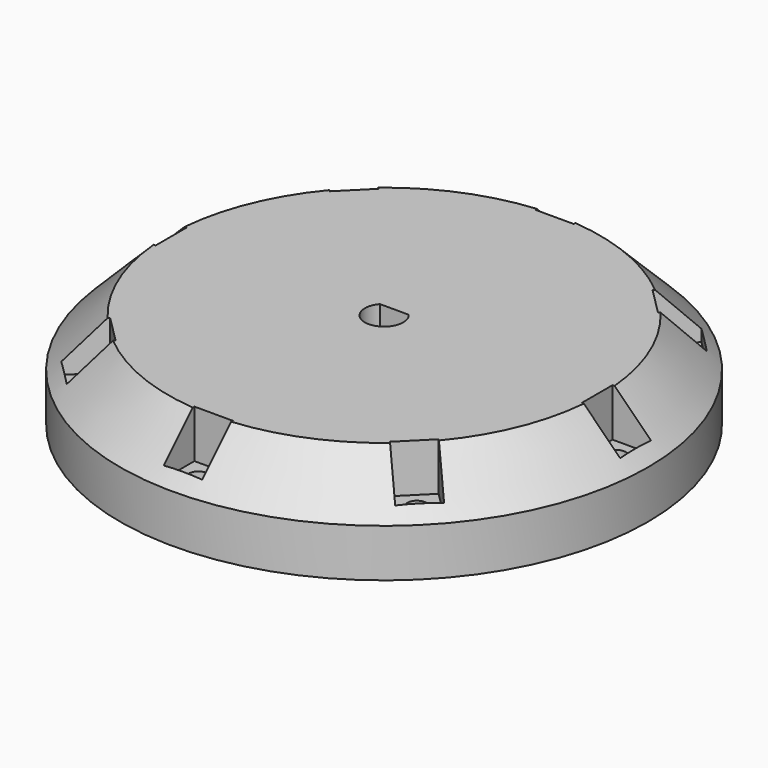
from build123d import *

# Parameters (mm, degrees)
F0_R     = 27.5
F0_R_2   = 1
F0_R_3   = 21.1
F1_DEPTH = 10
F3_DEPTH = 10
F5_W     = 4
F5_H     = 4
F5_R     = 1
F6_DEPTH = 5


# Not quite as in the source:
# - a fillet or chamfer that OpenCascade refuses, or shapes differently, is made with other operations: its cross-section is extruded or revolved along the edge and cut away or added


with BuildPart() as f1:
    # F0 (on Top) → F1 (new body)
    with BuildSketch(Plane.XY):
        Circle(F0_R)
        with Locations((-17.1119841047, -17.1119841047)):
            Circle(F0_R_2, mode=Mode.SUBTRACT)
        with Locations((0, -24.2)):
            Circle(F0_R_2, mode=Mode.SUBTRACT)
        with Locations((17.1119841047, -17.1119841047)):
            Circle(F0_R_2, mode=Mode.SUBTRACT)
        with Locations((-24.2, 0)):
            Circle(F0_R_2, mode=Mode.SUBTRACT)
        with Locations((-17.1119841047, 17.1119841047)):
            Circle(F0_R_2, mode=Mode.SUBTRACT)
        Circle(F0_R_3, mode=Mode.SUBTRACT)
        with Locations((24.2, 0)):
            Circle(F0_R_2, mode=Mode.SUBTRACT)
        with Locations((0, 24.2)):
            Circle(F0_R_2, mode=Mode.SUBTRACT)
        with Locations((17.1119841047, 17.1119841047)):
            Circle(F0_R_2, mode=Mode.SUBTRACT)
        Circle(F0_R_3)
        with BuildLine():
            ThreePointArc((1.4936867141, 1.33), (0, -2), (-1.4936867141, 1.33))
            Line((-1.4936867141, 1.33), (1.4936867141, 1.33))
        make_face(mode=Mode.SUBTRACT)
    extrude(amount=F1_DEPTH)

    # F2: chamfer of 5 on 1 edges, made by hand

    # F2_s1 → F2_t2 (revolve, cut)
    with BuildSketch(Plane.XZ):
        Polygon((27.5, 5), (22.5, 10), (27.5, 10), align=None)
    revolve(axis=Axis((0, 0, 10), (0, 0, 1)), mode=Mode.SUBTRACT)

    # F0 (on Top) → F3 (cut)
    with BuildSketch(Plane.XY):
        with BuildLine():
            Line((1.4936867141, 1.33), (-1.4936867141, 1.33))
            ThreePointArc((-1.4936867141, 1.33), (0, -2), (1.4936867141, 1.33))
        make_face()
    extrude(amount=F3_DEPTH, mode=Mode.SUBTRACT)

    # F5 (on offset) → F6 (cut)
    with BuildSketch(Plane.XY.offset(5)):
        with Locations((0, 24.2)):
            Rectangle(F5_W, F5_H)
        with Locations((0, 24.2)):
            Circle(F5_R, mode=Mode.SUBTRACT)
        with Locations((0, 24.2)):
            Circle(F5_R)
        Polygon((-14.28355698, 17.1119841047), (-17.1119841047, 19.9404112295), (-19.9404112295, 17.1119841047), (-17.1119841047, 14.28355698), align=None)
        Polygon((17.1119841047, 14.28355698), (19.9404112295, 17.1119841047), (17.1119841047, 19.9404112295), (14.28355698, 17.1119841047), align=None)
        with Locations((-24.2, 0)):
            Rectangle(F5_W, F5_H)
        Polygon((-17.1119841047, -14.28355698), (-19.9404112295, -17.1119841047), (-17.1119841047, -19.9404112295), (-14.28355698, -17.1119841047), align=None)
        with Locations((0, -24.2)):
            Rectangle(F5_W, F5_H)
        Polygon((14.28355698, -17.1119841047), (17.1119841047, -19.9404112295), (19.9404112295, -17.1119841047), (17.1119841047, -14.28355698), align=None)
        with Locations((24.2, 0)):
            Rectangle(F5_W, F5_H)
    extrude(amount=F6_DEPTH, mode=Mode.SUBTRACT)


solid = f1.part
